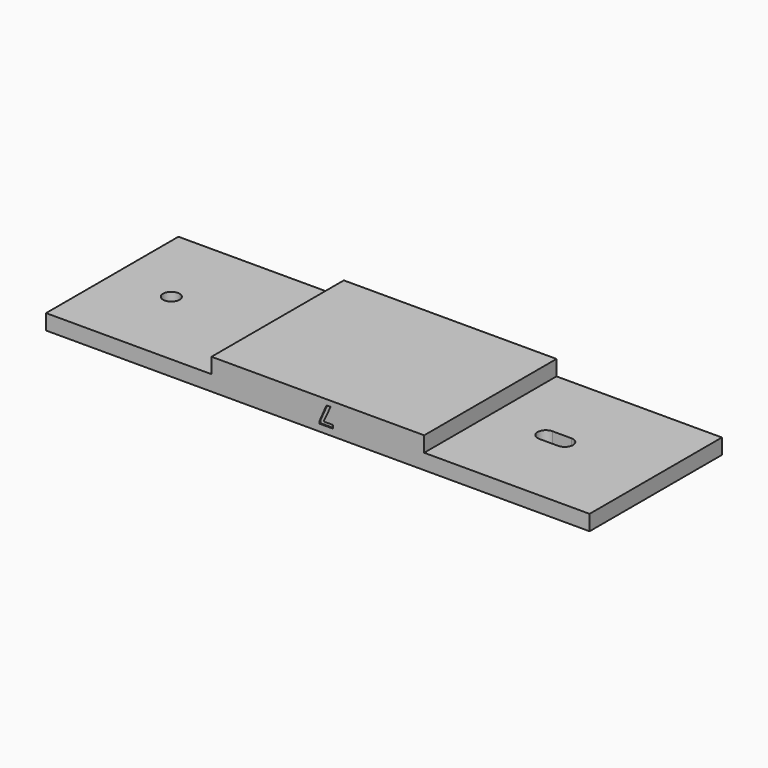
from build123d import *

# Parameters (mm, degrees)
F0_W           = 230
F0_H           = 70
F1_DEPTH       = 13
F4_W           = 70
F4_H           = 70
F5_DEPTH       = 6.5
F6_D           = 7
F6_CSINK_D     = 10
F6_CSINK_ANGLE = 90
F8_DEPTH       = 25
F9_TEXT_SIZE   = 10.9447884218
F10_DEPTH      = 0.5


# Not quite as in the source:
# - Text() gives the source's letters only with a copy of the font that has no kerning and outlines rounded to 1/6400 em; it was checked with that copy


with BuildPart() as f1:
    # F0 (on Top) → F1 (new body)
    with BuildSketch(Plane.XY):
        Rectangle(F0_W, F0_H)
    extrude(amount=F1_DEPTH)

    # F4 (on face) → F5 (cut)
    with BuildSketch(Plane.XY.offset(13)):
        with Locations((-80, 0)):
            Rectangle(F4_W, F4_H)
        with Locations((80, 0)):
            Rectangle(F4_W, F4_H)
    extrude(amount=-F5_DEPTH, mode=Mode.SUBTRACT)

    # F6 (through all)
    with Locations(Plane(origin=(0, 0, 0), x_dir=(1, 0, 0), z_dir=(0, 0, -1))):
        with Locations((-90, 0)):
            CounterSinkHole(F6_D / 2, F6_CSINK_D / 2, counter_sink_angle=F6_CSINK_ANGLE)

    # F7 (on face) → F8 (cut)
    with BuildSketch(Plane(origin=(0, 0, 0), x_dir=(1, 0, 0), z_dir=(0, 0, -1))):
        with BuildLine():
            ThreePointArc((68.5, 3.5), (65, 0), (68.5, -3.5))
            Line((68.5, -3.5), (76.5, -3.5))
            ThreePointArc((76.5, -3.5), (80, 0), (76.5, 3.5))
            Line((76.5, 3.5), (68.5, 3.5))
        make_face()
    extrude(amount=-F8_DEPTH, mode=Mode.SUBTRACT)

    # F9 (on face) → F10 (cut)
    with BuildSketch(Plane.XZ.offset(35)):
        with Locations(Location((6.6096261236, 10.7238527853), (0, 0, 180))):
            Text('7', F9_TEXT_SIZE, font='Open Sans', font_style=FontStyle.BOLD, text_align=(TextAlign.LEFT, TextAlign.BOTTOM))
    extrude(amount=-F10_DEPTH, mode=Mode.SUBTRACT)


solid = f1.part
